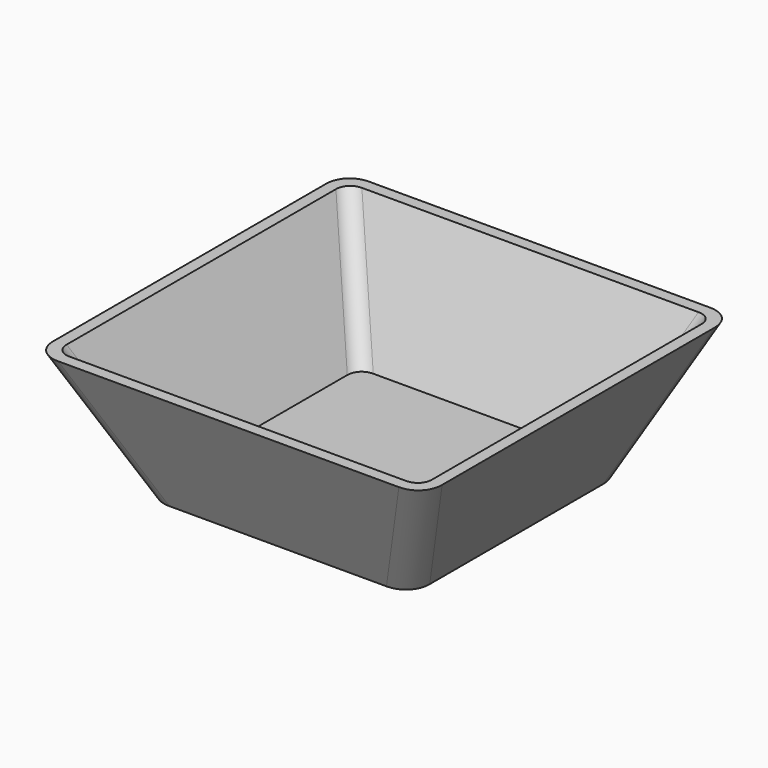
from build123d import *

# Parameters (mm, degrees)
F0_W                   = 50
F0_H                   = 50
F1_DEPTH               = 25
DRAFT_F1_DRAFTED_ANGLE = -25
F2_R                   = 5
F3_T                   = -2


# Not quite as in the source:
# - an extrude with a draft is written as a straight extrude whose walls are then drafted
# - the program builds the solid bodies; features that only make, move or delete a surface that nothing else refers to are left out


with BuildPart() as f1:
    # F0 (on Top) → F1 (new body)
    with BuildSketch(Plane.XY):
        Rectangle(F0_W, F0_H)
    extrude(amount=F1_DEPTH)

    # draft_F1_drafted
    draft_f1_drafted_walls = [f1.faces().sort_by_distance(p)[0] for p in [
        (0, -25, 16.6666666667),
        (25, 0, 16.6666666667),
        (0, 25, 16.6666666667),
        (-25, 0, 16.6666666667),
    ]]
    draft(draft_f1_drafted_walls, neutral_plane=Plane.XY, angle=DRAFT_F1_DRAFTED_ANGLE)

    # F2
    f2_edges = [f1.edges().sort_by_distance(p)[0] for p in [
        (-30.828846, -30.828846, 12.5),
        (30.828846, -30.828846, 12.5),
        (30.828846, 30.828846, 12.5),
        (-30.828846, 30.828846, 12.5),
    ]]
    fillet(f2_edges, radius=F2_R)

    # F3
    f3_openings = [f1.faces().sort_by_distance(p)[0] for p in [
        (0, 0, 25),
    ]]
    offset(amount=F3_T, openings=f3_openings)


solid = f1.part
